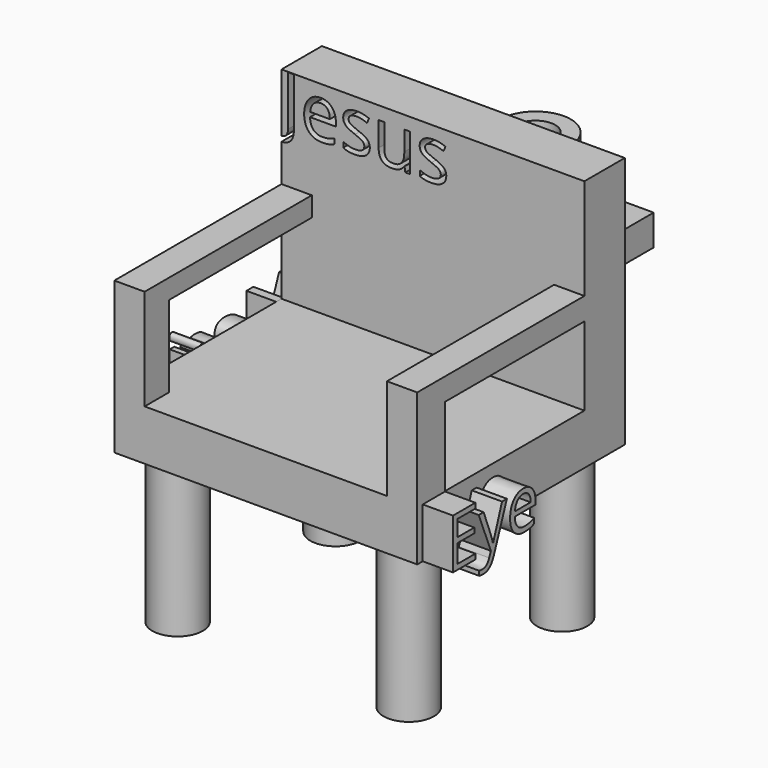
from build123d import *

# Parameters (mm, degrees)
F0_W          = 38.1
F0_H          = 32.6362870193
F1_DEPTH      = 6.35
F2_W          = 38.1
F2_H          = 6.35
F3_DEPTH      = 25.4
F4_R          = 3.175
F5_DEPTH      = 19.05
F6_R          = 3.175
F7_DEPTH      = 19.05
F8_R          = 3.175
F9_DEPTH      = 19.05
F10_R         = 3.175
F11_DEPTH     = 19.05
F12_W         = 3.81
F12_H         = 3.7967174433
F13_DEPTH     = 12.7
F14_W         = 3.81
F14_H         = 4.3750211376
F15_DEPTH     = 12.7
F16_W         = 3.81
F16_H         = 2.4754086018
F17_DEPTH     = 25.4
F18_W         = 3.81
F18_H         = 2.8166675448
F19_DEPTH     = 25.4
F20_TEXT_SIZE = 8.8194444444
F21_DEPTH     = 27.2813364863
F22_TEXT_SIZE = 8.8194444444
F23_DEPTH     = 3.81
F24_TEXT_SIZE = 8.8194444444
F25_DEPTH     = 3.81
F26_W         = 17.3677112907
F26_H         = 3.8693151027
F27_DEPTH     = 16.51
F28_R         = 4.4284694594
F29_DEPTH     = 8.89
F30_R         = 2.4804217363
F31_DEPTH     = 3.81
F32_TEXT_SIZE = 5.6163803404
F33_DEPTH     = 1.27
F34_TEXT_SIZE = 6.4740497078
F35_DEPTH     = 1.27
F36_TEXT_SIZE = 6.4739055491
F37_DEPTH     = 1.27
F38_TEXT_SIZE = 6.695839181
F39_DEPTH     = 1.27


# Not quite as in the source:
# - Text() gives the source's letters only with a copy of the font that has no kerning and outlines rounded to 1/6400 em; it was checked with that copy


with BuildPart() as f1:
    # F0 (on Top) → F1 (new body)
    with BuildSketch(Plane.XY):
        with Locations((0.2292171121, 11.943122372)):
            Rectangle(F0_W, F0_H)
    extrude(amount=F1_DEPTH)

    # F2 (on face) → F3 (join)
    with BuildSketch(Plane.XY.offset(6.35)):
        with Locations((0.2292171121, 25.0862658817)):
            Rectangle(F2_W, F2_H)
    extrude(amount=F3_DEPTH)

    # F4 (on face) → F5 (join)
    with BuildSketch(Plane(origin=(0, 0, 0), x_dir=(1, 0, 0), z_dir=(0, 0, -1))):
        with Locations((-14.3665699263, 0)):
            Circle(F4_R)
    extrude(amount=F5_DEPTH)

    # F6 (on face) → F7 (join)
    with BuildSketch(Plane(origin=(0, 0, 0), x_dir=(1, 0, 0), z_dir=(0, 0, -1))):
        with Locations((14.7134923958, 0)):
            Circle(F6_R)
    extrude(amount=F7_DEPTH)

    # F8 (on face) → F9 (join)
    with BuildSketch(Plane(origin=(0, 0, 0), x_dir=(1, 0, 0), z_dir=(0, 0, -1))):
        with Locations((-14.2277758569, -24.6652495116)):
            Circle(F8_R)
    extrude(amount=F9_DEPTH)

    # F10 (on face) → F11 (join)
    with BuildSketch(Plane(origin=(0, 0, 0), x_dir=(1, 0, 0), z_dir=(0, 0, -1))):
        with Locations((14.4942179322, -24.3920385838)):
            Circle(F10_R)
    extrude(amount=F11_DEPTH)

    # F12 (on face) → F13 (join)
    with BuildSketch(Plane.XY.offset(6.35)):
        with Locations((-16.9157828879, -2.476662416)):
            Rectangle(F12_W, F12_H)
    extrude(amount=F13_DEPTH)

    # F14 (on face) → F15 (join)
    with BuildSketch(Plane.XY.offset(6.35)):
        with Locations((17.3742171121, -2.1875105688)):
            Rectangle(F14_W, F14_H)
    extrude(amount=F15_DEPTH)

    # F16 (on face) → F17 (join)
    with BuildSketch(Plane(origin=(0, -0.5783036943, 0), x_dir=(-1, 0, 0), z_dir=(0, 1, 0))):
        with Locations((16.9157828879, 17.8122956991)):
            Rectangle(F16_W, F16_H)
    extrude(amount=F17_DEPTH)

    # F18 (on face) → F19 (join)
    with BuildSketch(Plane(origin=(0, 0, 0), x_dir=(-1, 0, 0), z_dir=(0, 1, 0))):
        with Locations((-17.3742171121, 17.6416662276)):
            Rectangle(F18_W, F18_H)
    extrude(amount=F19_DEPTH)

    # F20 (on face) → F21 (cut)
    with BuildSketch(Plane.XZ.offset(-21.9112658817)):
        with Locations((-18.8207828879, 25.4)):
            Text('Jesus', F20_TEXT_SIZE, font='Open Sans', text_align=(TextAlign.LEFT, TextAlign.BOTTOM))
    extrude(amount=-F21_DEPTH, mode=Mode.SUBTRACT)

    # F22 (on face) → F23 (join)
    with BuildSketch(Plane(origin=(-18.8207828879, 0, 0), x_dir=(0, -1, 0), z_dir=(-1, 0, 0))):
        with Locations((-28.2612658817, 0)):
            Text('Magic', F22_TEXT_SIZE, font='Open Sans', text_align=(TextAlign.LEFT, TextAlign.BOTTOM))
    extrude(amount=F23_DEPTH)

    # F24 (on face) → F25 (join)
    with BuildSketch(Plane.YZ.offset(19.2792171121)):
        with Locations((-4.3750211376, 0)):
            Text('Eye', F24_TEXT_SIZE, font='Open Sans', text_align=(TextAlign.LEFT, TextAlign.BOTTOM))
    extrude(amount=F25_DEPTH)

    # F26 (on face) → F27 (join)
    with BuildSketch(Plane(origin=(0, 28.2612658817, 0), x_dir=(-1, 0, 0), z_dir=(0, 1, 0))):
        with Locations((-1.0210676119, 13.9403424487)):
            Rectangle(F26_W, F26_H)
    extrude(amount=F27_DEPTH)

    # F28 (on face) → F29 (join)
    with BuildSketch(Plane.XY.offset(15.875)):
        with Locations((0.6341449916, 37.5361070037)):
            Circle(F28_R)
    extrude(amount=F29_DEPTH)

    # F30 (on face) → F31 (cut)
    with BuildSketch(Plane.XY.offset(24.765)):
        with Locations((0.6341449916, 37.5361070037)):
            Circle(F30_R)
    extrude(amount=-F31_DEPTH, mode=Mode.SUBTRACT)

    # F32 (on face) → F33 (cut)
    with BuildSketch(Plane(origin=(0, 0, -19.05), x_dir=(1, 0, 0), z_dir=(0, 0, -1))):
        with Locations((-16.5727575357, -26.5685560463)):
            Text('M', F32_TEXT_SIZE, font='Open Sans', text_align=(TextAlign.LEFT, TextAlign.BOTTOM))
    extrude(amount=-F33_DEPTH, mode=Mode.SUBTRACT)

    # F34 (on face) → F35 (cut)
    with BuildSketch(Plane(origin=(0, 0, -19.05), x_dir=(1, 0, 0), z_dir=(0, 0, -1))):
        with Locations((-16.553415583, -2.3595053992)):
            Text('C', F34_TEXT_SIZE, font='Open Sans', text_align=(TextAlign.LEFT, TextAlign.BOTTOM))
    extrude(amount=-F35_DEPTH, mode=Mode.SUBTRACT)

    # F36 (on face) → F37 (cut)
    with BuildSketch(Plane(origin=(0, 0, -19.05), x_dir=(1, 0, 0), z_dir=(0, 0, -1))):
        with Locations((12.3037573486, -26.7548799755)):
            Text('C', F36_TEXT_SIZE, font='Open Sans', text_align=(TextAlign.LEFT, TextAlign.BOTTOM))
    extrude(amount=-F37_DEPTH, mode=Mode.SUBTRACT)

    # F38 (on face) → F39 (cut)
    with BuildSketch(Plane(origin=(0, 0, -19.05), x_dir=(1, 0, 0), z_dir=(0, 0, -1))):
        with Locations((12.4148311233, -2.6308486555)):
            Text('T', F38_TEXT_SIZE, font='Open Sans', text_align=(TextAlign.LEFT, TextAlign.BOTTOM))
    extrude(amount=-F39_DEPTH, mode=Mode.SUBTRACT)


solid = f1.part
